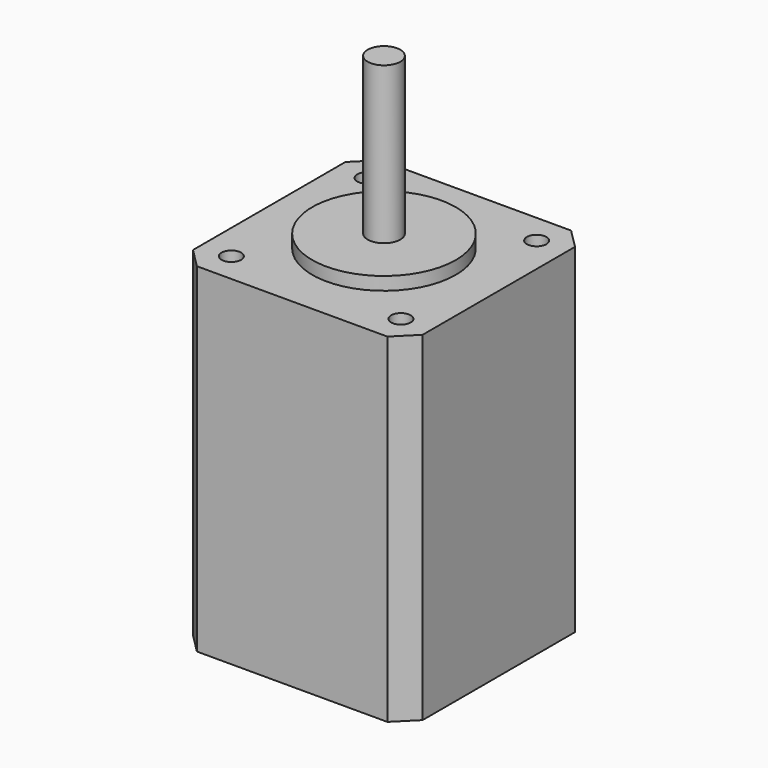
from build123d import *

# Parameters (mm, degrees)
F0_W     = 35.2
F0_H     = 35.2
F1_DEPTH = 52
F2_SIZE  = 3
F3_R     = 11
F4_DEPTH = 2
F5_R     = 2.5
F6_DEPTH = 24
F7_R     = 1.5
F8_DEPTH = 10


# Not quite as in the source:
# - a feature names something its author has since deleted; it is built from what else it names


with BuildPart() as f1:
    # F0 (on Top) → F1 (new body)
    with BuildSketch(Plane.XY):
        with Locations((17.6, 17.6)):
            Rectangle(F0_W, F0_H)
    extrude(amount=F1_DEPTH)

    # F2
    f2_edges = [f1.edges().sort_by_distance(p)[0] for p in [
        (0, 0, 26),
        (0, 35.2, 26),
        (35.2, 0, 26),
        (35.2, 35.2, 26),
    ]]
    chamfer(f2_edges, length=F2_SIZE)

    # F3 (on face) → F4 (join)
    with BuildSketch(Plane.XY.offset(52)):
        with Locations((17.6, 17.6)):
            Circle(F3_R)
    extrude(amount=F4_DEPTH)

    # F5 (on face) → F6 (join)
    with BuildSketch(Plane.XY.offset(54)):
        with Locations((17.6, 17.6)):
            Circle(F5_R)
    extrude(amount=F6_DEPTH)

    # F7 (on face) → F8 (cut)
    with BuildSketch(Plane.XY.offset(52)):
        with Locations((4.6, 30.6)):
            Circle(F7_R)
        with Locations((4.6, 4.6)):
            Circle(F7_R)
        with Locations((30.6, 30.6)):
            Circle(F7_R)
        with Locations((30.6, 4.6)):
            Circle(F7_R)
    extrude(amount=-F8_DEPTH, mode=Mode.SUBTRACT)


solid = f1.part
